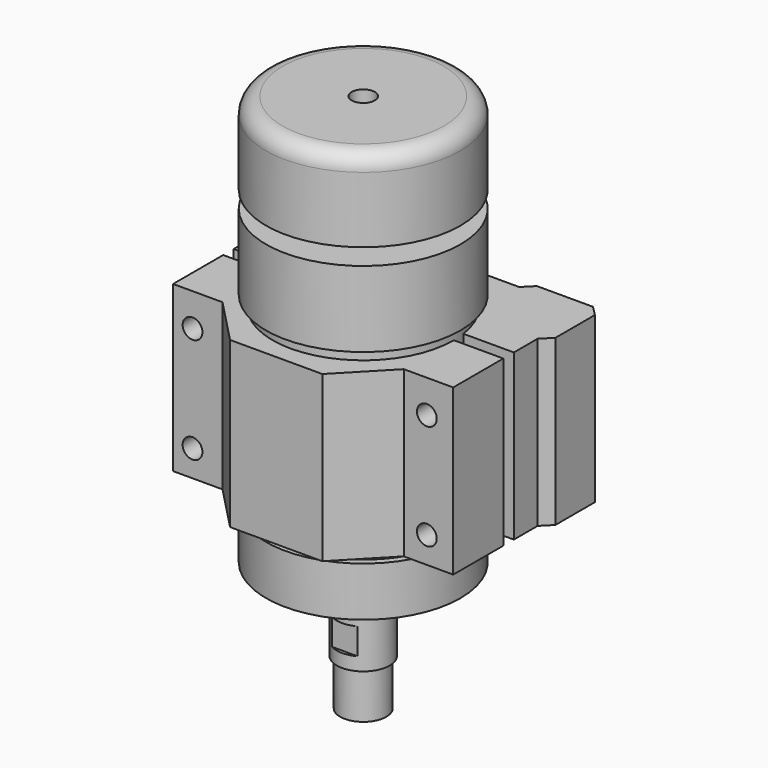
from build123d import *

# Parameters (mm, degrees)
F1_DEPTH      = 28.25
F2_R          = 29.5
F3_DEPTH      = 23
F4_R          = 29.5
F5_DEPTH      = 15
F6_R          = 12.5
F7_DEPTH      = 2
F8_R          = 3.5
F9_DEPTH      = 20
F9_DEPTH_BACK = 120
F11_R         = 8
F11_R_2       = 3.5
F12_DEPTH     = 20
F13_W         = 5.3180262744
F13_H         = 8
F14_DEPTH     = 5
F15_R         = 7
F15_R_2       = 5
F16_DEPTH     = 14
F18_R         = 3.5
F19_DEPTH     = 20
F20_R         = 29.5
F21_DEPTH     = 1.5
F22_R         = 29.5
F23_DEPTH     = 25
F24_R         = 5
F25_DEPTH     = 25
F27_D         = 6
F27_2_D       = 6


with BuildPart() as f1:
    # F0 (on Top) → F1 (new body, symmetric)
    with BuildSketch(Plane.XY):
        with BuildLine():
            ThreePointArc((-27.5, 0), (0, -27.5), (27.5, 0))
            ThreePointArc((27.5, 0), (27.4267864716, 2.0053388339), (27.2075357208, 4))
            ThreePointArc((27.2075357208, 4), (0, 27.5), (-27.2075357208, 4))
            ThreePointArc((-27.2075357208, 4), (-27.4267864716, 2.0053388339), (-27.5, 0))
        make_face()
    extrude(amount=F1_DEPTH, both=True)

    # F2 (on face) → F3 (join)
    with BuildSketch(Plane.XY.offset(28.25)):
        Circle(F2_R)
        with BuildLine():
            ThreePointArc((-27.5, 0), (-27.4267864716, 2.0053388339), (-27.2075357208, 4))
            ThreePointArc((-27.2075357208, 4), (0, 27.5), (27.2075357208, 4))
            ThreePointArc((27.2075357208, 4), (27.4267864716, 2.0053388339), (27.5, 0))
            ThreePointArc((27.5, 0), (0, -27.5), (-27.5, 0))
        make_face(mode=Mode.SUBTRACT)
        with BuildLine():
            ThreePointArc((27.2075357208, 4), (0, 27.5), (-27.2075357208, 4))
            ThreePointArc((-27.2075357208, 4), (-27.4267864716, 2.0053388339), (-27.5, 0))
            ThreePointArc((-27.5, 0), (0, -27.5), (27.5, 0))
            ThreePointArc((27.5, 0), (27.4267864716, 2.0053388339), (27.2075357208, 4))
        make_face()
    extrude(amount=F3_DEPTH)

    # F4 (on face) → F5 (join)
    with BuildSketch(Plane(origin=(0, 0, -28.25), x_dir=(1, 0, 0), z_dir=(0, 0, -1))):
        Circle(F4_R)
        with BuildLine():
            ThreePointArc((-27.2075357208, -4), (-27.4267864716, -2.0053388339), (-27.5, 0))
            ThreePointArc((-27.5, 0), (0, 27.5), (27.5, 0))
            ThreePointArc((27.5, 0), (27.4267864716, -2.0053388339), (27.2075357208, -4))
            ThreePointArc((27.2075357208, -4), (0, -27.5), (-27.2075357208, -4))
        make_face(mode=Mode.SUBTRACT)
        with BuildLine():
            ThreePointArc((27.5, 0), (0, 27.5), (-27.5, 0))
            ThreePointArc((-27.5, 0), (-27.4267864716, -2.0053388339), (-27.2075357208, -4))
            ThreePointArc((-27.2075357208, -4), (0, -27.5), (27.2075357208, -4))
            ThreePointArc((27.2075357208, -4), (27.4267864716, -2.0053388339), (27.5, 0))
        make_face()
    extrude(amount=F5_DEPTH)

    # F6 (on face) → F7 (join)
    with BuildSketch(Plane(origin=(0, 0, -43.25), x_dir=(1, 0, 0), z_dir=(0, 0, -1))):
        Circle(F6_R)
    extrude(amount=F7_DEPTH)

    # F8 (on face) → F9 (join, two sides)
    with BuildSketch(Plane(origin=(0, 0, -45.25), x_dir=(1, 0, 0), z_dir=(0, 0, -1))) as f9_sk:
        Circle(F8_R)
    extrude(amount=F9_DEPTH)
    extrude(f9_sk.sketch, amount=-F9_DEPTH_BACK)

    # F11 (on offset) → F12 (join)
    with BuildSketch(Plane(origin=(0, 0, -48.25), x_dir=(1, 0, 0), z_dir=(0, 0, -1))):
        Circle(F11_R)
        Circle(F11_R_2, mode=Mode.SUBTRACT)
    extrude(amount=F12_DEPTH)

    # F13 (on Right) → F14 (cut, symmetric)
    with BuildSketch(Plane.YZ):
        with Locations((9.6590131372, -60.25)):
            Rectangle(F13_W, F13_H)
        with Locations((-9.6590131372, -60.25)):
            Rectangle(F13_W, F13_H)
    extrude(amount=F14_DEPTH, both=True, mode=Mode.SUBTRACT)

    # F15 (on face) → F16 (join)
    with BuildSketch(Plane(origin=(0, 0, -68.25), x_dir=(1, 0, 0), z_dir=(0, 0, -1))):
        Circle(F15_R)
        Circle(F15_R_2, mode=Mode.SUBTRACT)
    extrude(amount=F16_DEPTH)

    # F18 (on offset) → F19 (join)
    with BuildSketch(Plane.XY.offset(61.25)):
        with BuildLine():
            Line((-0.5, -5.4772255751), (-0.5, -29.1325048873))
            Line((-0.5, -29.1325048873), (0.5, -29.1325048873))
            Line((0.5, -29.1325048873), (0.5, -5.4772255751))
            ThreePointArc((0.5, -5.4772255751), (1.6995934691, -5.2308108396), (2.8149239193, -4.7250611984))
            Line((2.8149239193, -4.7250611984), (16.7191482379, -23.8625841687))
            Line((16.7191482379, -23.8625841687), (17.5281652323, -23.2747989164))
            Line((17.5281652323, -23.2747989164), (3.6239409137, -4.1372759461))
            ThreePointArc((3.6239409137, -4.1372759461), (4.4495934691, -3.2328188876), (5.0546425772, -2.1680840429))
            Line((5.0546425772, -2.1680840429), (27.5521501119, -9.477967357))
            Line((27.5521501119, -9.477967357), (27.8611671063, -8.5269108407))
            Line((27.8611671063, -8.5269108407), (5.3636595716, -1.2170275266))
            ThreePointArc((5.3636595716, -1.2170275266), (5.5, 0), (5.3636595716, 1.2170275266))
            Line((5.3636595716, 1.2170275266), (27.8611671063, 8.5269108407))
            Line((27.8611671063, 8.5269108407), (27.5521501119, 9.477967357))
            Line((27.5521501119, 9.477967357), (5.0546425772, 2.1680840429))
            ThreePointArc((5.0546425772, 2.1680840429), (4.4495934691, 3.2328188876), (3.6239409137, 4.1372759461))
            Line((3.6239409137, 4.1372759461), (17.5281652323, 23.2747989164))
            Line((17.5281652323, 23.2747989164), (16.7191482379, 23.8625841687))
            Line((16.7191482379, 23.8625841687), (2.8149239193, 4.7250611984))
            ThreePointArc((2.8149239193, 4.7250611984), (1.6995934691, 5.2308108396), (0.5, 5.4772255751))
            Line((0.5, 5.4772255751), (0.5, 29.1325048873))
            Line((0.5, 29.1325048873), (-0.5, 29.1325048873))
            Line((-0.5, 29.1325048873), (-0.5, 5.4772255751))
            ThreePointArc((-0.5, 5.4772255751), (-1.6995934691, 5.2308108396), (-2.8149239193, 4.7250611984))
            Line((-2.8149239193, 4.7250611984), (-16.7191482379, 23.8625841687))
            Line((-16.7191482379, 23.8625841687), (-17.5281652323, 23.2747989164))
            Line((-17.5281652323, 23.2747989164), (-3.6239409137, 4.1372759461))
            ThreePointArc((-3.6239409137, 4.1372759461), (-4.4495934691, 3.2328188876), (-5.0546425772, 2.1680840429))
            Line((-5.0546425772, 2.1680840429), (-27.5521501119, 9.477967357))
            Line((-27.5521501119, 9.477967357), (-27.8611671063, 8.5269108407))
            Line((-27.8611671063, 8.5269108407), (-5.3636595716, 1.2170275266))
            ThreePointArc((-5.3636595716, 1.2170275266), (-5.5, 0), (-5.3636595716, -1.2170275266))
            Line((-5.3636595716, -1.2170275266), (-27.8611671063, -8.5269108407))
            Line((-27.8611671063, -8.5269108407), (-27.5521501119, -9.477967357))
            Line((-27.5521501119, -9.477967357), (-5.0546425772, -2.1680840429))
            ThreePointArc((-5.0546425772, -2.1680840429), (-4.4495934691, -3.2328188876), (-3.6239409137, -4.1372759461))
            Line((-3.6239409137, -4.1372759461), (-17.5281652323, -23.2747989164))
            Line((-17.5281652323, -23.2747989164), (-16.7191482379, -23.8625841687))
            Line((-16.7191482379, -23.8625841687), (-2.8149239193, -4.7250611984))
            ThreePointArc((-2.8149239193, -4.7250611984), (-1.6995934691, -5.2308108396), (-0.5, -5.4772255751))
        make_face()
        Circle(F18_R, mode=Mode.SUBTRACT)
    extrude(amount=F19_DEPTH)

    # F20 (on face) → F21 (join)
    with BuildSketch(Plane.XY.offset(81.25)):
        Circle(F20_R)
        with BuildLine():
            ThreePointArc((-0.5, -5.4772255751), (-1.6995934691, -5.2308108396), (-2.8149239193, -4.7250611984))
            Line((-2.8149239193, -4.7250611984), (-16.7191482379, -23.8625841687))
            Line((-16.7191482379, -23.8625841687), (-17.5281652323, -23.2747989164))
            Line((-17.5281652323, -23.2747989164), (-3.6239409137, -4.1372759461))
            ThreePointArc((-3.6239409137, -4.1372759461), (-4.4495934691, -3.2328188876), (-5.0546425772, -2.1680840429))
            Line((-5.0546425772, -2.1680840429), (-27.5521501119, -9.477967357))
            Line((-27.5521501119, -9.477967357), (-27.8611671063, -8.5269108407))
            Line((-27.8611671063, -8.5269108407), (-5.3636595716, -1.2170275266))
            ThreePointArc((-5.3636595716, -1.2170275266), (-5.5, 0), (-5.3636595716, 1.2170275266))
            Line((-5.3636595716, 1.2170275266), (-27.8611671063, 8.5269108407))
            Line((-27.8611671063, 8.5269108407), (-27.5521501119, 9.477967357))
            Line((-27.5521501119, 9.477967357), (-5.0546425772, 2.1680840429))
            ThreePointArc((-5.0546425772, 2.1680840429), (-4.4495934691, 3.2328188876), (-3.6239409137, 4.1372759461))
            Line((-3.6239409137, 4.1372759461), (-17.5281652323, 23.2747989164))
            Line((-17.5281652323, 23.2747989164), (-16.7191482379, 23.8625841687))
            Line((-16.7191482379, 23.8625841687), (-2.8149239193, 4.7250611984))
            ThreePointArc((-2.8149239193, 4.7250611984), (-1.6995934691, 5.2308108396), (-0.5, 5.4772255751))
            Line((-0.5, 5.4772255751), (-0.5, 29.1325048873))
            Line((-0.5, 29.1325048873), (0.5, 29.1325048873))
            Line((0.5, 29.1325048873), (0.5, 5.4772255751))
            ThreePointArc((0.5, 5.4772255751), (1.6995934691, 5.2308108396), (2.8149239193, 4.7250611984))
            Line((2.8149239193, 4.7250611984), (16.7191482379, 23.8625841687))
            Line((16.7191482379, 23.8625841687), (17.5281652323, 23.2747989164))
            Line((17.5281652323, 23.2747989164), (3.6239409137, 4.1372759461))
            ThreePointArc((3.6239409137, 4.1372759461), (4.4495934691, 3.2328188876), (5.0546425772, 2.1680840429))
            Line((5.0546425772, 2.1680840429), (27.5521501119, 9.477967357))
            Line((27.5521501119, 9.477967357), (27.8611671063, 8.5269108407))
            Line((27.8611671063, 8.5269108407), (5.3636595716, 1.2170275266))
            ThreePointArc((5.3636595716, 1.2170275266), (5.5, 0), (5.3636595716, -1.2170275266))
            Line((5.3636595716, -1.2170275266), (27.8611671063, -8.5269108407))
            Line((27.8611671063, -8.5269108407), (27.5521501119, -9.477967357))
            Line((27.5521501119, -9.477967357), (5.0546425772, -2.1680840429))
            ThreePointArc((5.0546425772, -2.1680840429), (4.4495934691, -3.2328188876), (3.6239409137, -4.1372759461))
            Line((3.6239409137, -4.1372759461), (17.5281652323, -23.2747989164))
            Line((17.5281652323, -23.2747989164), (16.7191482379, -23.8625841687))
            Line((16.7191482379, -23.8625841687), (2.8149239193, -4.7250611984))
            ThreePointArc((2.8149239193, -4.7250611984), (1.6995934691, -5.2308108396), (0.5, -5.4772255751))
            Line((0.5, -5.4772255751), (0.5, -29.1325048873))
            Line((0.5, -29.1325048873), (-0.5, -29.1325048873))
            Line((-0.5, -29.1325048873), (-0.5, -5.4772255751))
        make_face(mode=Mode.SUBTRACT)
    extrude(amount=-F21_DEPTH)

    # F22 (on face) → F23 (join)
    with BuildSketch(Plane.XY.offset(81.25)):
        Circle(F22_R)
        with BuildLine():
            ThreePointArc((26.7587528212, 8.1687147261), (27.6879173769, 4.1312405775), (28, 0))
            ThreePointArc((28, 0), (27.6879173769, -4.1312405775), (26.7587528212, -8.1687147261))
            Line((26.7587528212, -8.1687147261), (27.8611671063, -8.5269108407))
            Line((27.8611671063, -8.5269108407), (27.5521501119, -9.477967357))
            Line((27.5521501119, -9.477967357), (26.4443913566, -9.1180347188))
            ThreePointArc((26.4443913566, -9.1180347188), (22.5825116788, -16.3894074926), (16.7412512355, -22.1917047183))
            Line((16.7412512355, -22.1917047183), (17.5281652323, -23.2747989164))
            Line((17.5281652323, -23.2747989164), (16.7191482379, -23.8625841687))
            Line((16.7191482379, -23.8625841687), (15.9235859071, -22.76758656))
            ThreePointArc((15.9235859071, -22.76758656), (8.5666402424, -26.2902893708), (0.5, -27.5))
            Line((0.5, -27.5), (0.5, -29.1325048873))
            Line((0.5, -29.1325048873), (-0.5, -29.1325048873))
            Line((-0.5, -29.1325048873), (-0.5, -27.4818121673))
            ThreePointArc((-0.5, -27.4818121673), (-8.4270223583, -26.0107337808), (-15.5867427383, -22.3039617124))
            Line((-15.5867427383, -22.3039617124), (-16.7191482379, -23.8625841687))
            Line((-16.7191482379, -23.8625841687), (-17.5281652323, -23.2747989164))
            Line((-17.5281652323, -23.2747989164), (-16.3871113987, -21.7042730495))
            ThreePointArc((-16.3871113987, -21.7042730495), (-21.9111509737, -15.9370735091), (-25.5452273296, -8.8258786163))
            Line((-25.5452273296, -8.8258786163), (-27.5521501119, -9.477967357))
            Line((-27.5521501119, -9.477967357), (-27.8611671063, -8.5269108407))
            Line((-27.8611671063, -8.5269108407), (-25.8488998538, -7.8730855763))
            ThreePointArc((-25.8488998538, -7.8730855763), (-27, 0), (-25.8488998538, 7.8730855763))
            Line((-25.8488998538, 7.8730855763), (-27.8611671063, 8.5269108407))
            Line((-27.8611671063, 8.5269108407), (-27.5521501119, 9.477967357))
            Line((-27.5521501119, 9.477967357), (-25.5452273296, 8.8258786163))
            ThreePointArc((-25.5452273296, 8.8258786163), (-21.9111509737, 15.9370735091), (-16.3871113987, 21.7042730495))
            Line((-16.3871113987, 21.7042730495), (-17.5281652323, 23.2747989164))
            Line((-17.5281652323, 23.2747989164), (-16.7191482379, 23.8625841687))
            Line((-16.7191482379, 23.8625841687), (-15.5867427383, 22.3039617124))
            ThreePointArc((-15.5867427383, 22.3039617124), (-8.4270223583, 26.0107337808), (-0.5, 27.4818121673))
            Line((-0.5, 27.4818121673), (-0.5, 29.1325048873))
            Line((-0.5, 29.1325048873), (0.5, 29.1325048873))
            Line((0.5, 29.1325048873), (0.5, 27.5))
            ThreePointArc((0.5, 27.5), (8.5666402424, 26.2902893708), (15.9235859071, 22.76758656))
            Line((15.9235859071, 22.76758656), (16.7191482379, 23.8625841687))
            Line((16.7191482379, 23.8625841687), (17.5281652323, 23.2747989164))
            Line((17.5281652323, 23.2747989164), (16.7412512355, 22.1917047183))
            ThreePointArc((16.7412512355, 22.1917047183), (22.5825116788, 16.3894074926), (26.4443913566, 9.1180347188))
            Line((26.4443913566, 9.1180347188), (27.5521501119, 9.477967357))
            Line((27.5521501119, 9.477967357), (27.8611671063, 8.5269108407))
            Line((27.8611671063, 8.5269108407), (26.7587528212, 8.1687147261))
        make_face(mode=Mode.SUBTRACT)
        with BuildLine():
            ThreePointArc((-25.8488998538, 7.8730855763), (-25.7013948956, 8.3508625619), (-25.5452273296, 8.8258786163))
            Line((-25.5452273296, 8.8258786163), (-27.5521501119, 9.477967357))
            Line((-27.5521501119, 9.477967357), (-27.8611671063, 8.5269108407))
            Line((-27.8611671063, 8.5269108407), (-25.8488998538, 7.8730855763))
        make_face()
        with BuildLine():
            Line((-27.5521501119, -9.477967357), (-25.5452273296, -8.8258786163))
            ThreePointArc((-25.5452273296, -8.8258786163), (-25.7013948956, -8.3508625619), (-25.8488998538, -7.8730855763))
            Line((-25.8488998538, -7.8730855763), (-27.8611671063, -8.5269108407))
            Line((-27.8611671063, -8.5269108407), (-27.5521501119, -9.477967357))
        make_face()
        with BuildLine():
            ThreePointArc((-16.3871113987, 21.7042730495), (-15.9896534465, 22.0077561149), (-15.5867427383, 22.3039617124))
            Line((-15.5867427383, 22.3039617124), (-16.7191482379, 23.8625841687))
            Line((-16.7191482379, 23.8625841687), (-17.5281652323, 23.2747989164))
            Line((-17.5281652323, 23.2747989164), (-16.3871113987, 21.7042730495))
        make_face()
        with BuildLine():
            Line((-16.7191482379, -23.8625841687), (-15.5867427383, -22.3039617124))
            ThreePointArc((-15.5867427383, -22.3039617124), (-15.9896534465, -22.0077561149), (-16.3871113987, -21.7042730495))
            Line((-16.3871113987, -21.7042730495), (-17.5281652323, -23.2747989164))
            Line((-17.5281652323, -23.2747989164), (-16.7191482379, -23.8625841687))
        make_face()
        with BuildLine():
            ThreePointArc((-0.5, 27.4818121673), (-8.26925e-05, 27.4954526659), (0.5, 27.5))
            Line((0.5, 27.5), (0.5, 29.1325048873))
            Line((0.5, 29.1325048873), (-0.5, 29.1325048873))
            Line((-0.5, 29.1325048873), (-0.5, 27.4818121673))
        make_face()
        with BuildLine():
            Line((0.5, -29.1325048873), (0.5, -27.5))
            ThreePointArc((0.5, -27.5), (-8.26925e-05, -27.4954526659), (-0.5, -27.4818121673))
            Line((-0.5, -27.4818121673), (-0.5, -29.1325048873))
            Line((-0.5, -29.1325048873), (0.5, -29.1325048873))
        make_face()
        with BuildLine():
            ThreePointArc((15.9235859071, 22.76758656), (16.3350367158, 22.4833630093), (16.7412512355, 22.1917047183))
            Line((16.7412512355, 22.1917047183), (17.5281652323, 23.2747989164))
            Line((17.5281652323, 23.2747989164), (16.7191482379, 23.8625841687))
            Line((16.7191482379, 23.8625841687), (15.9235859071, 22.76758656))
        make_face()
        with BuildLine():
            Line((17.5281652323, -23.2747989164), (16.7412512355, -22.1917047183))
            ThreePointArc((16.7412512355, -22.1917047183), (16.3350367158, -22.4833630093), (15.9235859071, -22.76758656))
            Line((15.9235859071, -22.76758656), (16.7191482379, -23.8625841687))
            Line((16.7191482379, -23.8625841687), (17.5281652323, -23.2747989164))
        make_face()
        with BuildLine():
            ThreePointArc((26.4443913566, 9.1180347188), (26.6058876046, 8.6448037789), (26.7587528212, 8.1687147261))
            Line((26.7587528212, 8.1687147261), (27.8611671063, 8.5269108407))
            Line((27.8611671063, 8.5269108407), (27.5521501119, 9.477967357))
            Line((27.5521501119, 9.477967357), (26.4443913566, 9.1180347188))
        make_face()
        with BuildLine():
            Line((27.8611671063, -8.5269108407), (26.7587528212, -8.1687147261))
            ThreePointArc((26.7587528212, -8.1687147261), (26.6058876046, -8.6448037789), (26.4443913566, -9.1180347188))
            Line((26.4443913566, -9.1180347188), (27.5521501119, -9.477967357))
            Line((27.5521501119, -9.477967357), (27.8611671063, -8.5269108407))
        make_face()
    extrude(amount=-F23_DEPTH)

    # F24
    f24_edges = [f1.edges().sort_by_distance(p)[0] for p in [
        (-29.5, 0, 81.25),
    ]]
    fillet(f24_edges, radius=F24_R)


with BuildPart() as f25:
    # F0 (on Top) → F25 (new body, symmetric)
    with BuildSketch(Plane.XY):
        with BuildLine():
            Line((42.5, 0), (27.5, 0))
            ThreePointArc((27.5, 0), (0, -27.5), (-27.5, 0))
            Line((-27.5, 0), (-42.5, 0))
            Line((-42.5, 0), (-42.5, -19))
            Line((-42.5, -19), (-27.5, -19))
            Line((-27.5, -19), (-14, -33))
            Line((-14, -33), (0, -33))
            Line((0, -33), (14, -33))
            Line((14, -33), (27.5, -19))
            Line((27.5, -19), (42.5, -19))
            Line((42.5, -19), (42.5, 0))
        make_face()
    extrude(amount=F25_DEPTH, both=True)

    # F27 (through all)
    with Locations(Plane.XZ.offset(19)):
        with Locations((-36.6, 15), (-36.6, -17), (34.5, 15), (34.5, -17)):
            Hole(F27_D / 2)


with BuildPart() as f25b:
    # F0 (on Top) → F25, piece 2 (new body, symmetric)
    with BuildSketch(Plane.XY):
        with BuildLine():
            ThreePointArc((-27.2075357208, 4), (0, 27.5), (27.2075357208, 4))
            Line((27.2075357208, 4), (42.5, 4))
            Line((42.5, 4), (42.5, 13))
            Line((42.5, 13), (45.5, 16))
            Line((45.5, 16), (45.5, 31))
            Line((45.5, 31), (42.5, 34))
            Line((42.5, 34), (25.5, 34))
            Line((25.5, 34), (22.5, 31))
            Line((22.5, 31), (10, 31))
            Line((10, 31), (7, 34))
            Line((7, 34), (0, 34))
            Line((0, 34), (-7, 34))
            Line((-7, 34), (-10, 31))
            Line((-10, 31), (-22.5, 31))
            Line((-22.5, 31), (-25.5, 34))
            Line((-25.5, 34), (-42.5, 34))
            Line((-42.5, 34), (-45.5, 31))
            Line((-45.5, 31), (-45.5, 16))
            Line((-45.5, 16), (-42.5, 13))
            Line((-42.5, 13), (-42.5, 4))
            Line((-42.5, 4), (-27.2075357208, 4))
        make_face()
    extrude(amount=F25_DEPTH, both=True)

    # F27#2 (through all)
    with Locations(Plane.XZ.offset(19)):
        with Locations((-36.6, 15), (-36.6, -17), (34.5, 15), (34.5, -17)):
            Hole(F27_2_D / 2)


solid = Compound([f1.part, f25.part, f25b.part])
